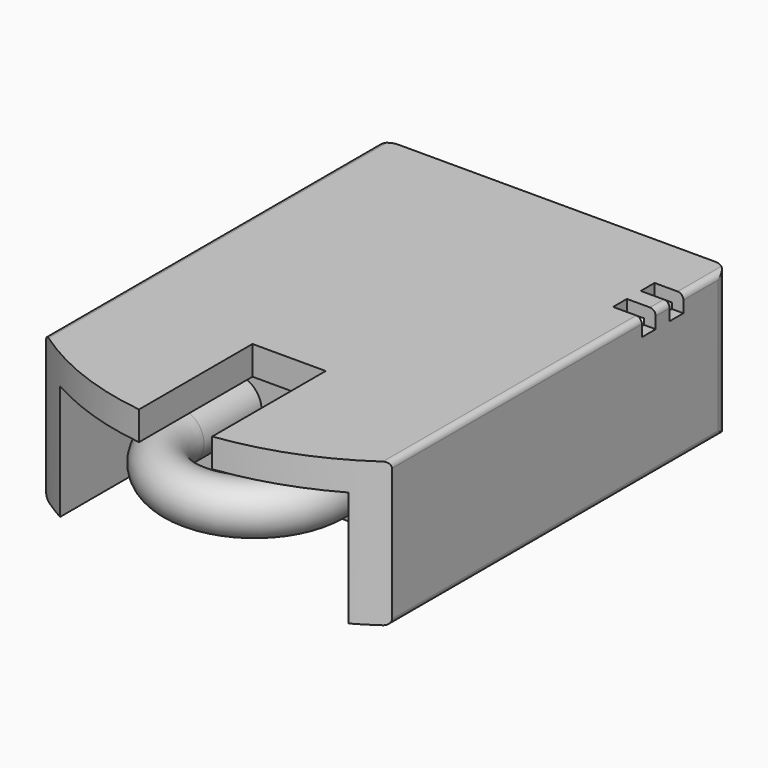
from build123d import *

# Parameters (mm, degrees)
F1_DEPTH    = 25
F3_R        = 2.54
F4_W        = 50
F4_H        = 30
F5_DEPTH    = 20
F2_W        = 12.7
F2_H        = 25
F6_DEPTH    = 25
F7_T        = -2
F8_T1_DEPTH = 75.655609521
F10_W       = 5
F10_H       = 15
F11_DEPTH   = 10
F12_W       = 7.3
F12_H       = 11.5
F13_DEPTH   = 25.4
F16_R       = 4.25
F18_W       = 5
F18_H       = 3
F19_DEPTH   = 3


# Not quite as in the source:
# - a fillet or chamfer that OpenCascade refuses, or shapes differently, is made with other operations: its cross-section is extruded or revolved along the edge and cut away or added
# - a feature names something its author has since deleted; it is built from what else it names


with BuildPart() as f1:
    # F0 (on Top) → F1 (new body)
    with BuildSketch(Plane.XY):
        with BuildLine():
            Line((30, -36.5978047605), (30, 36.5978047605))
            Line((30, 36.5978047605), (-30, 36.5978047605))
            Line((-30, 36.5978047605), (-30, -36.5978047605))
            ThreePointArc((-30, -36.5978047605), (0, -46.4021952395), (30, -36.5978047605))
        make_face()
    extrude(amount=F1_DEPTH)

    # F3
    f3_edges = [f1.edges().sort_by_distance(p)[0] for p in [
        (-30, 36.597805, 12.5),
        (30, 36.597805, 12.5),
    ]]
    fillet(f3_edges, radius=F3_R)

    # F4 (on face) → F5 (cut)
    with BuildSketch(Plane.XY):
        with Locations((0, -31.4021952395)):
            Rectangle(F4_W, F4_H)
    extrude(amount=F5_DEPTH, mode=Mode.SUBTRACT)

    # F2 (on Top) → F6 (cut, through all)
    with BuildSketch(Plane.XY):
        with Locations((0, -33.9021952395)):
            Rectangle(F2_W, F2_H)
    extrude(amount=F6_DEPTH, mode=Mode.SUBTRACT)

    # F7 (hollow: no face is removed)
    offset(amount=F7_T, kind=Kind.INTERSECTION, mode=Mode.SUBTRACT)

    # F8: fillet of radius 1 on 4 edges, made by hand

    # F8_s2 → F8_t1 (cut)
    with BuildSketch(Plane.XZ.offset(-36.5578047605)):
        with BuildLine():
            ThreePointArc((29, 0), (29.7071067812, 0.2928932188), (30, 1))
            Line((30, 1), (30, 0))
            Line((30, 0), (29, 0))
        make_face()
        with BuildLine():
            ThreePointArc((29, 25), (29.7071067812, 24.7071067812), (30, 24))
            Line((30, 24), (30, 25))
            Line((30, 25), (29, 25))
        make_face()
        with BuildLine():
            ThreePointArc((-29, 25), (-29.7071067812, 24.7071067812), (-30, 24))
            Line((-30, 24), (-30, 25))
            Line((-30, 25), (-29, 25))
        make_face()
        with BuildLine():
            ThreePointArc((-29, 0), (-29.7071067812, 0.2928932188), (-30, 1))
            Line((-30, 1), (-30, 0))
            Line((-30, 0), (-29, 0))
        make_face()
    extrude(amount=F8_T1_DEPTH, mode=Mode.SUBTRACT)

    # F10 (on face) → F11 (cut)
    with BuildSketch(Plane(origin=(0, 36.5978047605, 0), x_dir=(-1, 0, 0), z_dir=(0, 1, 0))):
        with Locations((-15.5, 12.5)):
            Rectangle(F10_W, F10_H)
        with Locations((15.5, 12.5)):
            Rectangle(F10_W, F10_H)
        with Locations((-5.5, 12.5)):
            Rectangle(F10_W, F10_H)
        with Locations((5.5, 12.5)):
            Rectangle(F10_W, F10_H)
    extrude(amount=-F11_DEPTH, mode=Mode.SUBTRACT)

    # F12 (on face) → F13 (cut)
    with BuildSketch(Plane(origin=(0, 36.5978047605, 0), x_dir=(-1, 0, 0), z_dir=(0, 1, 0))):
        with Locations((23.35, 12.5)):
            Rectangle(F12_W, F12_H)
    extrude(amount=-F13_DEPTH, mode=Mode.SUBTRACT)

    # F17: sweep along a path in F15
    with BuildLine(Plane.XY.offset(12)) as f17_path:
        Line((-13, -16.4021952395), (-13, -28.9021952395))
        ThreePointArc((-13, -28.9021952395), (0, -41.9021952395), (13, -28.9021952395))
        Line((13, -28.9021952395), (13, -16.4021952395))
    # F16 (on face) → F17 (sweep)
    with BuildSketch(Plane.XZ.offset(16.4021952395)):
        with Locations((-13.0000123754, 11.9999870658)):
            Circle(F16_R)
    sweep(path=f17_path.line)

    # F18 (on face) → F19 (cut)
    with BuildSketch(Plane.XY.offset(25)):
        with Locations((27.5, 25.0978047605)):
            Rectangle(F18_W, F18_H)
        with Locations((27.5, 19.0978047605)):
            Rectangle(F18_W, F18_H)
    extrude(amount=-F19_DEPTH, mode=Mode.SUBTRACT)


solid = f1.part
